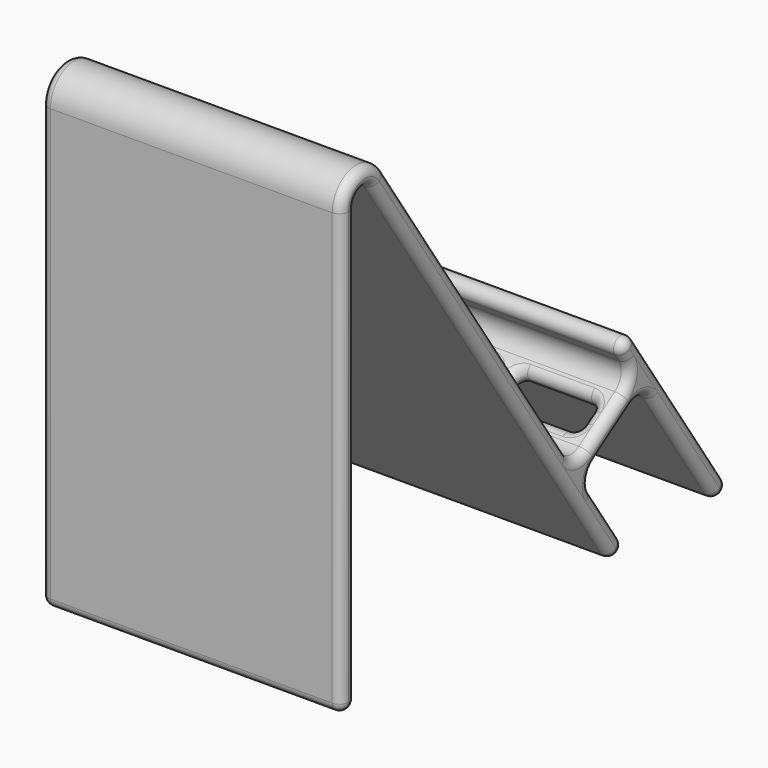
from build123d import *

# Parameters (mm, degrees)
F1_DEPTH = 25
F3_DEPTH = 32.001
F4_R     = 1.49999


# Not quite as in the source:
# - a fillet or chamfer is up to 0.001 mm smaller than in the source, because OpenCascade refuses the exact size


with BuildPart() as f1:
    # F0 (on Right) → F1 (new body, symmetric)
    with BuildSketch(Plane.YZ):
        with BuildLine():
            Line((-3.6055512755, 0), (0, 0))
            Line((0, 0), (-7.7658027472, 11.6487041207))
            ThreePointArc((-7.7658027472, 11.6487041207), (-8.2113938912, 13.9011531148), (-6.9337524528, 15.8089555924))
            Line((-6.9337524528, 15.8089555924), (0.5547001962, 20.8012573584))
            ThreePointArc((0.5547001962, 20.8012573584), (2.8071491903, 21.2468485025), (4.7149516679, 19.9692070641))
            Line((4.7149516679, 19.9692070641), (18.0277563773, 0))
            Line((18.0277563773, 0), (21.6333076528, 0))
            Line((21.6333076528, 0), (1.3867504906, 30.3698357433))
            ThreePointArc((1.3867504906, 30.3698357433), (0.4328492518, 31.0086564625), (-0.6933752453, 30.7858608905))
            ThreePointArc((-0.6933752453, 30.7858608905), (-1.3321959645, 29.8319596517), (-1.1094003925, 28.7057351547))
            Line((-1.1094003925, 28.7057351547), (-0.2773500981, 27.4576597131))
            ThreePointArc((-0.2773500981, 27.4576597131), (0.1682410459, 25.2052107191), (-1.1094003925, 23.2974082415))
            Line((-1.1094003925, 23.2974082415), (-8.5978530415, 18.3051064754))
            ThreePointArc((-8.5978530415, 18.3051064754), (-10.8503020356, 17.8595153314), (-12.7581045132, 19.1371567698))
            Line((-12.7581045132, 19.1371567698), (-50.8397485283, 76.2596227925))
            ThreePointArc((-50.8397485283, 76.2596227925), (-56.4489207434, 78.2715819438), (-60, 73.4861218113))
            Line((-60, 73.4861218113), (-60, 0))
            Line((-60, 0), (-57, 0))
            Line((-57, 0), (-57, 73.4861218113))
            ThreePointArc((-57, 73.4861218113), (-55.5795682974, 75.4003058643), (-53.3358994113, 74.5955222038))
            Line((-53.3358994113, 74.5955222038), (-3.6055512755, 0))
        make_face()
    extrude(amount=F1_DEPTH, both=True)

    # F2 (on face) → F3 (cut, through all)
    with BuildSketch(Plane(origin=(0, -11.0940039245, 16.6410058868), x_dir=(1, 0, 0), z_dir=(0, -0.5547001962, 0.8320502943))):
        with BuildLine():
            ThreePointArc((22, 8.5), (21.5606601718, 9.5606601718), (20.5, 10))
            Line((20.5, 10), (9.8333333333, 10))
            ThreePointArc((9.8333333333, 10), (8.7726731616, 9.5606601718), (8.3333333333, 8.5))
            Line((8.3333333333, 8.5), (8.3333333333, 6.5))
            ThreePointArc((8.3333333333, 6.5), (8.7726731616, 5.4393398282), (9.8333333333, 5))
            Line((9.8333333333, 5), (20.5, 5))
            ThreePointArc((20.5, 5), (21.5606601718, 5.4393398282), (22, 6.5))
            Line((22, 6.5), (22, 8.5))
        make_face()
        with BuildLine():
            ThreePointArc((3.8333333333, 5), (4.8939935051, 5.4393398282), (5.3333333333, 6.5))
            Line((5.3333333333, 6.5), (5.3333333333, 8.5))
            ThreePointArc((5.3333333333, 8.5), (4.8939935051, 9.5606601718), (3.8333333333, 10))
            Line((3.8333333333, 10), (-3.8333333333, 10))
            ThreePointArc((-3.8333333333, 10), (-4.8939935051, 9.5606601718), (-5.3333333333, 8.5))
            Line((-5.3333333333, 8.5), (-5.3333333333, 6.5))
            ThreePointArc((-5.3333333333, 6.5), (-4.8939935051, 5.4393398282), (-3.8333333333, 5))
            Line((-3.8333333333, 5), (3.8333333333, 5))
        make_face()
        with BuildLine():
            ThreePointArc((-22, 6.5), (-21.5606601718, 5.4393398282), (-20.5, 5))
            Line((-20.5, 5), (-9.8333333333, 5))
            ThreePointArc((-9.8333333333, 5), (-8.7726731616, 5.4393398282), (-8.3333333333, 6.5))
            Line((-8.3333333333, 6.5), (-8.3333333333, 8.5))
            ThreePointArc((-8.3333333333, 8.5), (-8.7726731616, 9.5606601718), (-9.8333333333, 10))
            Line((-9.8333333333, 10), (-20.5, 10))
            ThreePointArc((-20.5, 10), (-21.5606601718, 9.5606601718), (-22, 8.5))
            Line((-22, 8.5), (-22, 6.5))
        make_face()
    extrude(amount=-F3_DEPTH, mode=Mode.SUBTRACT)

    # F4 (radius 1.5 in the source; OpenCascade refuses exactly that, so slightly less here)
    f4_edges = [f1.edges().sort_by_distance(p)[0] for p in [
        (0, -1.1094, 23.297408),
        (-25, -4.853627, 20.801257),
        (25, -4.853627, 20.801257),
        (0, -8.597853, 18.305106),
        (-21.56066, -3.139054, 21.944306),
        (-22, -4.853627, 20.801257),
        (-21.56066, -6.5682, 19.658209),
        (-15.166667, -6.933752, 19.414507),
        (-8.772673, -6.5682, 19.658209),
        (-8.333333, -4.853627, 20.801257),
        (-8.772673, -3.139054, 21.944306),
        (-15.166667, -2.773501, 22.188008),
        (-4.893994, -6.5682, 19.658209),
        (0, -6.933752, 19.414507),
        (4.893994, -6.5682, 19.658209),
        (5.333333, -4.853627, 20.801257),
        (4.893994, -3.139054, 21.944306),
        (0, -2.773501, 22.188008),
        (-4.893994, -3.139054, 21.944306),
        (-5.333333, -4.853627, 20.801257),
        (21.56066, -6.5682, 19.658209),
        (22, -4.853627, 20.801257),
        (21.56066, -3.139054, 21.944306),
        (15.166667, -2.773501, 22.188008),
        (8.772673, -3.139054, 21.944306),
        (8.333333, -4.853627, 20.801257),
        (8.772673, -6.5682, 19.658209),
        (15.166667, -6.933752, 19.414507),
        (0, -6.933752, 15.808956),
        (-25, -3.189526, 18.305106),
        (25, -3.189526, 18.305106),
        (0, 0.5547, 20.801257),
        (-5.333333, -3.189526, 18.305106),
        (-4.893994, -1.474953, 19.448155),
        (0, -1.1094, 19.691857),
        (4.893994, -1.474953, 19.448155),
        (5.333333, -3.189526, 18.305106),
        (4.893994, -4.904099, 17.162058),
        (0, -5.269652, 16.918356),
        (-4.893994, -4.904099, 17.162058),
        (-15.166667, -1.1094, 19.691857),
        (-8.772673, -1.474953, 19.448155),
        (-8.333333, -3.189526, 18.305106),
        (-8.772673, -4.904099, 17.162058),
        (-15.166667, -5.269652, 16.918356),
        (-21.56066, -4.904099, 17.162058),
        (-22, -3.189526, 18.305106),
        (-21.56066, -1.474953, 19.448155),
        (15.166667, -5.269652, 16.918356),
        (8.772673, -4.904099, 17.162058),
        (8.333333, -3.189526, 18.305106),
        (8.772673, -1.474953, 19.448155),
        (15.166667, -1.1094, 19.691857),
        (21.56066, -1.474953, 19.448155),
        (22, -3.189526, 18.305106),
        (21.56066, -4.904099, 17.162058),
        (0, -53.335899, 74.595522),
        (-25, -28.470725, 37.297761),
        (0, -3.605551, 0),
        (25, -28.470725, 37.297761),
        (-25, -1.802776, 0),
        (0, 0, 0),
        (25, -1.802776, 0),
        (-25, 19.830532, 0),
        (0, 21.633308, 0),
        (25, 19.830532, 0),
        (0, 18.027756, 0),
        (0, -60, 0),
        (-25, -58.5, 0),
        (0, -57, 0),
        (25, -58.5, 0),
    ]]
    fillet(f4_edges, radius=F4_R)


solid = f1.part
